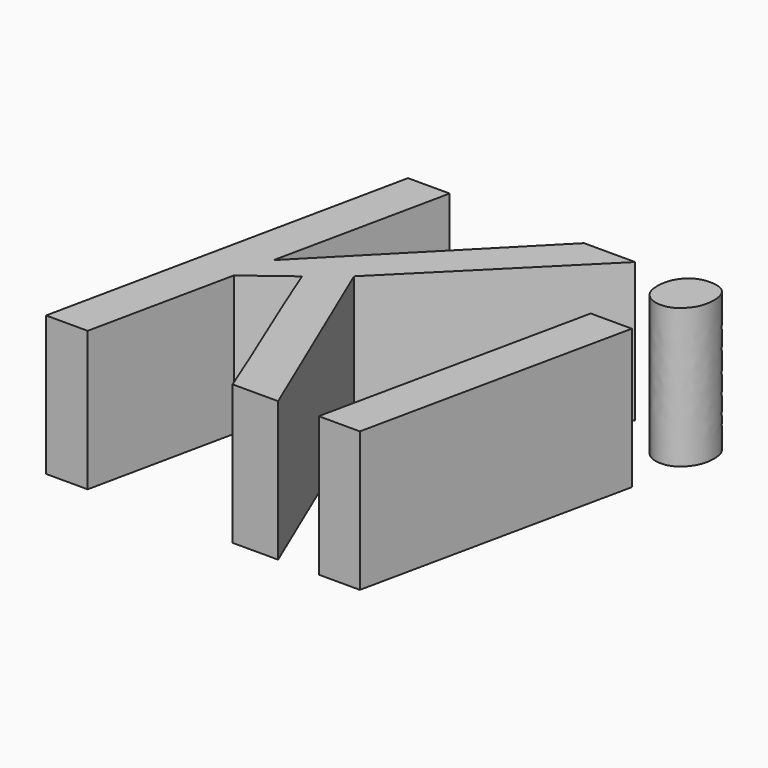
from build123d import *

# Parameters (mm, degrees)
F0_TEXT_SIZE = 35.9260994527
F1_DEPTH     = 10


# Not quite as in the source:
# - Text() gives the source's letters only with a copy of the font that has no kerning and outlines rounded to 1/6400 em; it was checked with that copy


with BuildPart() as f1:
    # F0 (on Top) → F1 (new body)
    with BuildSketch(Plane.XY):
        with Locations((-49.2906048894, 11.0652372241)):
            Text('Ki', F0_TEXT_SIZE, font='Open Sans', font_style=FontStyle.ITALIC, text_align=(TextAlign.LEFT, TextAlign.BOTTOM))
    extrude(amount=F1_DEPTH)


solid = f1.part
